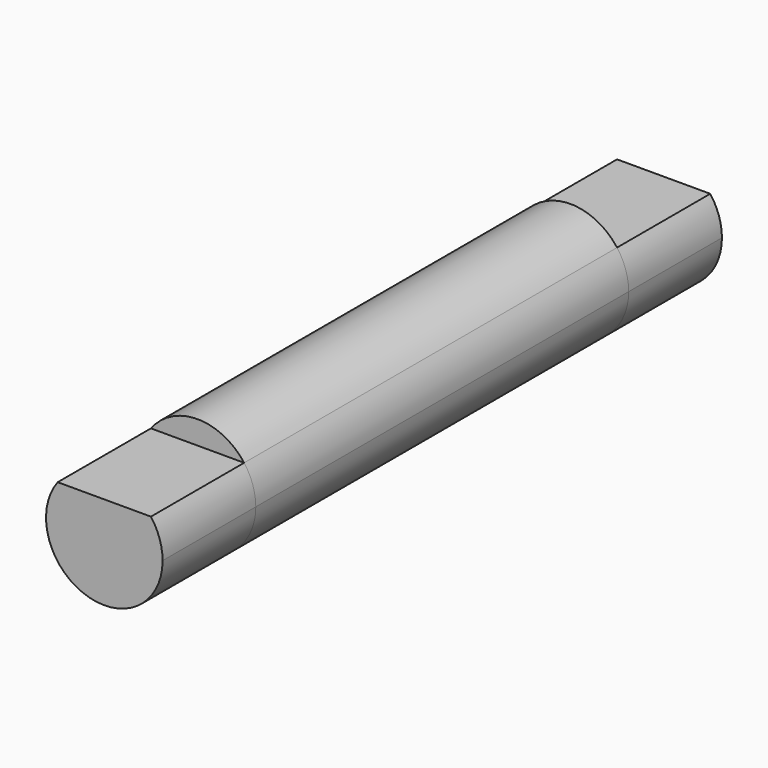
from build123d import *
from build123d import SkipClean  # not in build123d's __all__

# Parameters (mm, degrees)
F1_DEPTH = 30
F3_START = -5
F2_R     = 2.5
F3_DEPTH = 20


with BuildPart() as f1:
    # F0 (on Front) → F1 (new body)
    with BuildSketch(Plane.XZ):
        with BuildLine():
            ThreePointArc((-2, 1.5), (-0.790569415, -2.3717082451), (2.5, 0))
            ThreePointArc((2.5, 0), (2.3717082451, 0.790569415), (2, 1.5))
            Line((2, 1.5), (-2, 1.5))
        make_face()
    extrude(amount=F1_DEPTH)

    # F2 (on face) → F3 (join)
    with BuildSketch(Plane.XZ.offset(30).offset(F3_START)):
        Circle(F2_R)
    with SkipClean():  # cleaning this boolean's faces spoils the solid; the shape is the same uncleaned
        extrude(amount=-F3_DEPTH)


solid = f1.part
